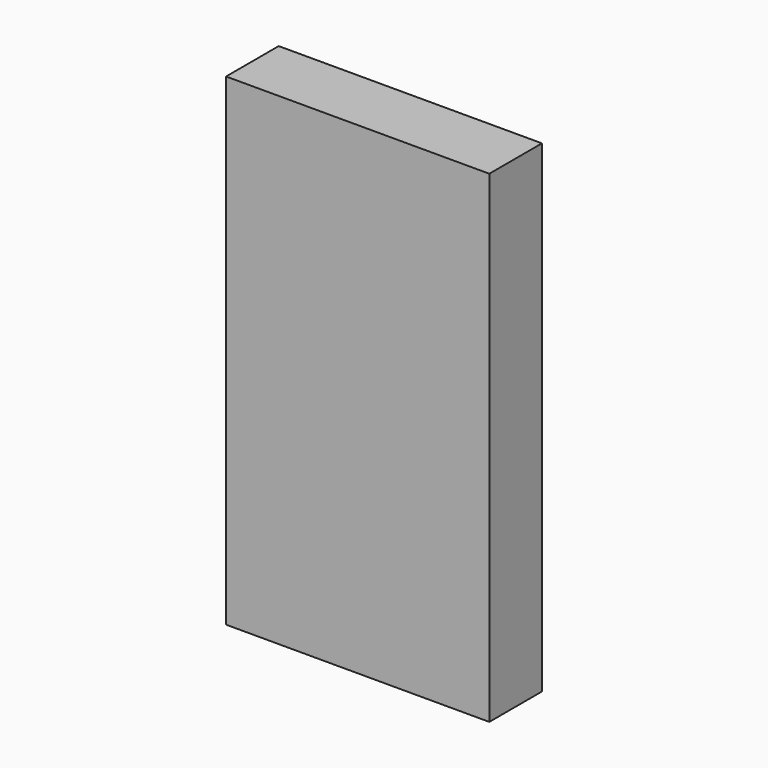
from build123d import *

# Parameters (mm, degrees)
F0_W     = 60
F0_H     = 15
F1_DEPTH = 110


# Not quite as in the source:
# - a feature names something its author has since deleted; it is built from what else it names


with BuildPart() as f1:
    # F0 (on Top) → F1 (new body)
    with BuildSketch(Plane.XY):
        Rectangle(F0_W, F0_H)
    extrude(amount=F1_DEPTH)


solid = f1.part
